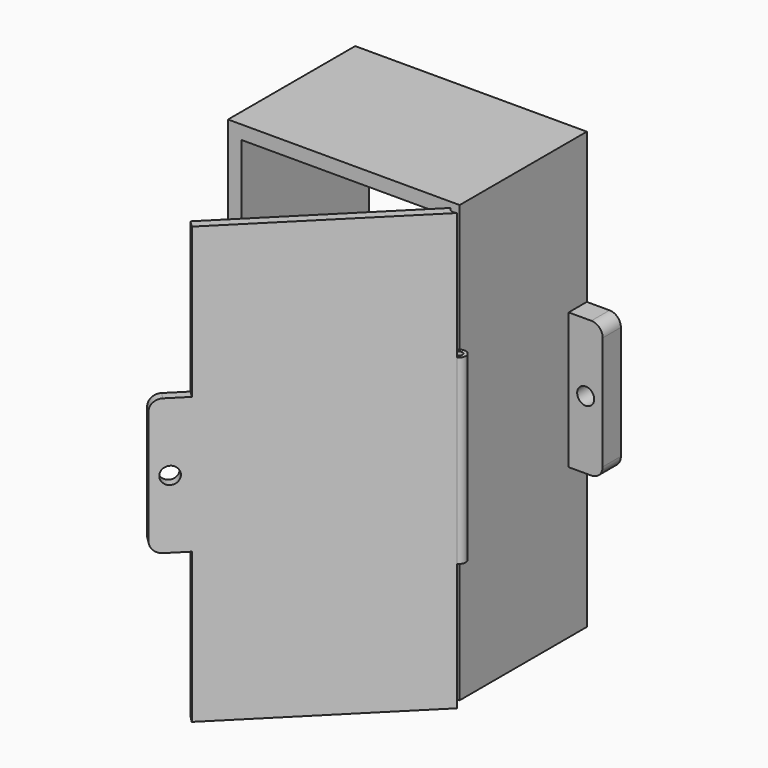
from build123d import *

# Parameters (mm, degrees)
F0_W           = 90
F0_H           = 180
F1_DEPTH       = 70
F0_W_2         = 15
F0_H_2         = 60
F0_R           = 3.75
F2_DEPTH       = 10
F3_R           = 5
F5_R           = 3
F5_R_2         = 1.5
F6_DEPTH       = 40
F7_W           = 15
F7_H           = 60
F7_R           = 3.75
F8_DEPTH       = 6
F11_END_RADIUS = 3
F10_W          = 4
F10_H          = 192
F11_REACH      = 324.2716302284
F12_R          = 3.75
F13_DEPTH      = 4
F14_R          = 5
F15_R          = 5


with BuildPart() as f1:
    # F0 (on Front) → F1 (new body)
    with BuildSketch(Plane.XZ):
        Polygon((51, 96), (-51, 96), (-51, 30), (-51, -30), (-51, -96), (51, -96), (51, -30), (51, 30), align=None)
        Rectangle(F0_W, F0_H, mode=Mode.SUBTRACT)
    extrude(amount=F1_DEPTH)

    # F0 (on Front) → F2 (join)
    with BuildSketch(Plane.XZ):
        with Locations((-58.5, 0)):
            Rectangle(F0_W_2, F0_H_2)
        with Locations((-58.5, 0)):
            Circle(F0_R, mode=Mode.SUBTRACT)
        with Locations((58.5, 0)):
            Rectangle(F0_W_2, F0_H_2)
        with Locations((58.5, 0)):
            Circle(F0_R, mode=Mode.SUBTRACT)
    extrude(amount=F2_DEPTH)

    # F3
    f3_edges = [f1.edges().sort_by_distance(p)[0] for p in [
        (66, -5, 30),
        (66, -5, -30),
        (-66, -5, -30),
        (-66, -5, 30),
    ]]
    fillet(f3_edges, radius=F3_R)


with BuildPart() as f6:
    # F5 (on Top) → F6 (new body, symmetric)
    with BuildSketch(Plane.XY):
        with Locations((52.6971285333, -72.4738138049)):
            Circle(F5_R)
        with Locations((52.6971285333, -72.4738138049)):
            Circle(F5_R_2, mode=Mode.SUBTRACT)
    extrude(amount=F6_DEPTH, both=True)

    f11_end = (Plane(origin=(52.6971285333, -72.4738138049, 0), x_dir=(1, 0, 0), z_dir=(0, 0, 1)) * Cylinder(F11_END_RADIUS, 1138.3770958347, mode=Mode.PRIVATE)).faces().sort_by_distance((49.6971285333, -72.4738138049, 0))[0]
    # F10 (on face) → F11 (join, up to the whole of a round face its end follows)
    with BuildSketch(Plane(origin=(-60.5, -60.5, 0), x_dir=(0.7071067812, -0.7071067812, 0), z_dir=(-0.7071067812, -0.7071067812, 0))):
        with Locations((89.3599205236, 0)):
            Rectangle(F10_W, F10_H)
    f11_long = extrude(amount=-F11_REACH, mode=Mode.PRIVATE)
    add(split(f11_long, bisect_by=f11_end, keep=Keep.ALL, mode=Mode.PRIVATE).solids().sort_by_distance((2.6870057685, -123.6870057685, 0))[0])

    # F12 (on face) → F13 (join)
    with BuildSketch(Plane(origin=(61.7727922061, -61.7727922061, 0), x_dir=(-0.7071067812, -0.7071067812, 0), z_dir=(-0.7071067812, 0.7071067812, 0))):
        Polygon((85.5599205236, 96), (85.5599205236, -96), (106.7553205236, -96), (106.7553205236, -30), (121.7553205236, -30), (121.7553205236, 30), (106.7553205236, 30), (106.7553205236, 96), align=None)
        with Locations((114.2553205236, 0)):
            Circle(F12_R, mode=Mode.SUBTRACT)
    extrude(amount=-F13_DEPTH)

    # F14
    f14_edges = [f6.edges().sort_by_distance(p)[0] for p in [
        (-22.907007, -149.281019, 30),
        (-22.907007, -149.281019, -30),
    ]]
    fillet(f14_edges, radius=F14_R)


with BuildPart() as f8:
    # F7 (on face) → F8 (new body)
    with BuildSketch(Plane.XZ.offset(70)):
        with Locations((-58.5, 0)):
            Rectangle(F7_W, F7_H)
        with Locations((-58.5, 0)):
            Circle(F7_R, mode=Mode.SUBTRACT)
    extrude(amount=-F8_DEPTH)

    # F15
    f15_edges = [f8.edges().sort_by_distance(p)[0] for p in [
        (-66, -67, 30),
        (-66, -67, -30),
    ]]
    fillet(f15_edges, radius=F15_R)


with BuildPart() as f6_1:
    # F16: moved
    add(f6.part)


solid = Compound([f1.part, f8.part, f6_1.part])
